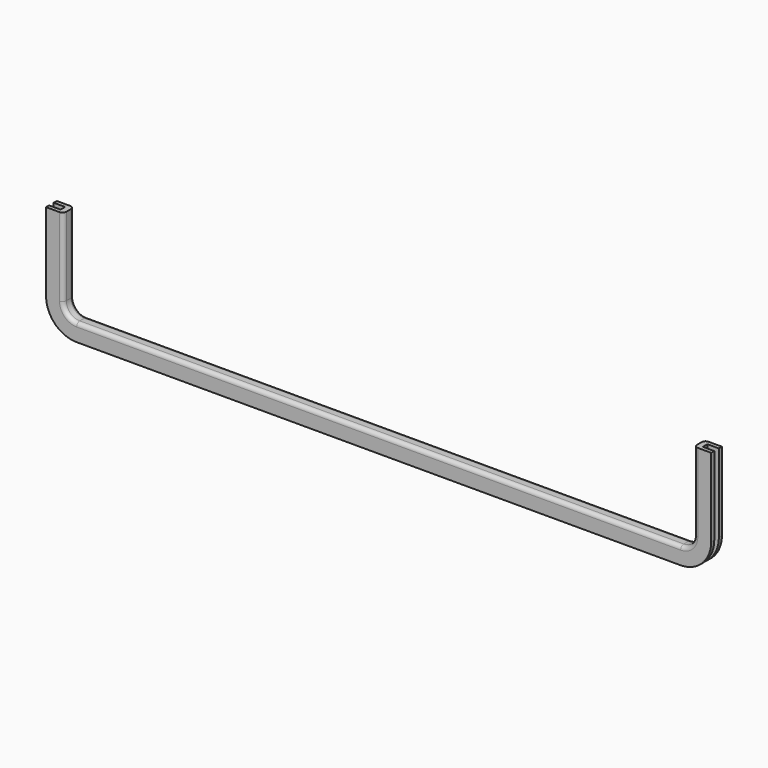
from build123d import *

# Parameters (mm, degrees)
F1_DEPTH = 1.5
F3_DEPTH = 1
F5_DEPTH = 1
F6_R     = 0.99999


# Not quite as in the source:
# - a fillet or chamfer is up to 0.001 mm smaller than in the source, because OpenCascade refuses the exact size
# - ends of sketch curves that miss each other by under 0.0002 mm in the source are joined


with BuildPart() as f1:
    # F0 (on Front) → F1 (new body)
    with BuildSketch(Plane.XZ):
        with BuildLine():
            Line((1.5, 25.5), (0, 25.5))
            Line((0, 25.5), (0, 5))
            ThreePointArc((0, 5), (1.4644660941, 1.4644660941), (5, 0))
            Line((5, 0), (163, 0))
            ThreePointArc((163, 0), (166.5355339059, 1.4644660941), (168, 5))
            Line((168, 5), (168, 25.5))
            Line((168, 25.5), (166.5, 25.5))
            Line((166.5, 25.5), (166.5, 5))
            ThreePointArc((166.5, 5), (165.4748737342, 2.5251262658), (163, 1.5))
            Line((163, 1.5), (5, 1.5))
            ThreePointArc((5, 1.5), (2.5251262658, 2.5251262658), (1.5, 5))
            Line((1.5, 5), (1.5, 25.5))
        make_face()
    extrude(amount=F1_DEPTH)

    # F2 (on face) → F3 (join)
    with BuildSketch(Plane.XZ.offset(1.5)):
        with BuildLine():
            Line((1.5, 5), (1.5, 25.5))
            Line((1.5, 25.5), (-3, 25.5))
            Line((-3, 25.5), (-3, 4.9999991791))
            ThreePointArc((-3, 4.9999991791), (-0.6568544899, -0.6568544899), (4.9999991791, -3))
            Line((4.9999991791, -3), (163, -3))
            ThreePointArc((163, -3), (168.6568542495, -0.6568542495), (171, 5))
            Line((171, 5), (171, 25.5))
            Line((171, 25.5), (166.5, 25.5))
            Line((166.5, 25.5), (166.5, 5))
            ThreePointArc((166.5, 5), (165.4748737342, 2.5251262658), (163, 1.5))
            Line((163, 1.5), (5, 1.5))
            ThreePointArc((5, 1.5), (2.5251257352, 2.5251263156), (1.5, 5))
        make_face()
    extrude(amount=F3_DEPTH)

    # F4 (on face) → F5 (join)
    with BuildSketch(Plane(origin=(0, 0, 0), x_dir=(-1, 0, 0), z_dir=(0, 1, 0))):
        with BuildLine():
            Line((-166.5, 5), (-166.5, 25.5))
            Line((-166.5, 25.5), (-171, 25.5))
            Line((-171, 25.5), (-171, 5))
            ThreePointArc((-171, 5), (-168.6568542495, -0.6568542495), (-163, -3))
            Line((-163, -3), (-5, -3))
            ThreePointArc((-5, -3), (0.6568542495, -0.6568542495), (3, 5))
            Line((3, 5), (3, 25.5))
            Line((3, 25.5), (-1.5, 25.5))
            Line((-1.5, 25.5), (-1.5, 5))
            ThreePointArc((-1.5, 5), (-2.5251262658, 2.5251262658), (-5, 1.5))
            Line((-5, 1.5), (-163, 1.5))
            ThreePointArc((-163, 1.5), (-165.4748737342, 2.5251262658), (-166.5, 5))
        make_face()
    extrude(amount=F5_DEPTH)

    # F6 (radius 1 in the source; OpenCascade refuses exactly that, so slightly less here)
    f6_edges = [f1.edges().sort_by_distance(p)[0] for p in [
        (165.474874, 1, 2.525126),
        (166.5, -2.5, 15.25),
    ]]
    fillet(f6_edges, radius=F6_R)


solid = f1.part
